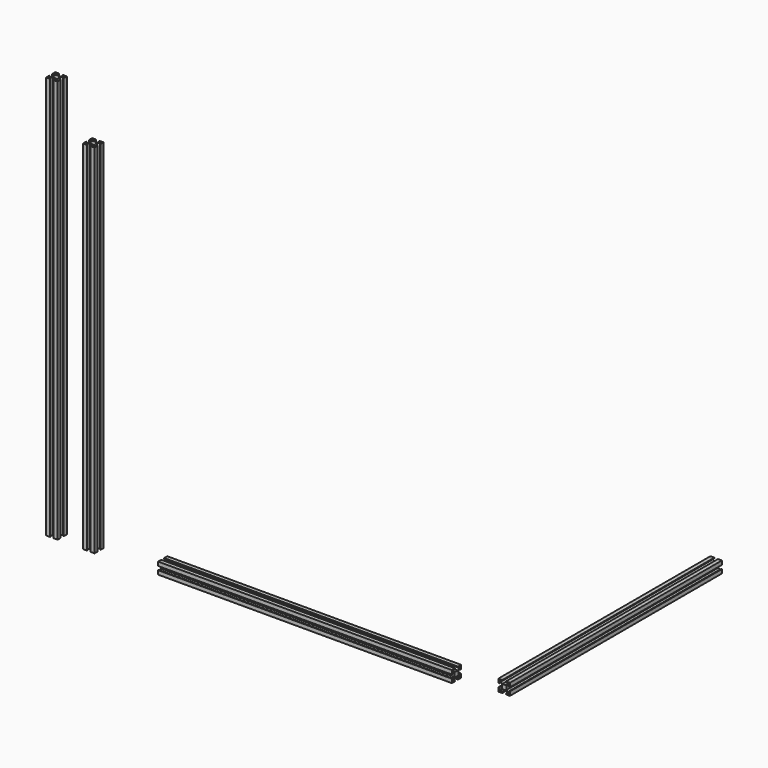
from build123d import *

# Parameters (mm, degrees)
F0_W     = 20
F0_H     = 700
F1_DEPTH = 20
F0_W_2   = 510
F0_H_2   = 20
F0_H_3   = 620
F2_DEPTH = 460
F4_DEPTH = 620
F6_DEPTH = 700
F8_DEPTH = 510


# Not quite as in the source:
# - a feature names something its author has since deleted; it is built from what else it names


with BuildPart() as f1:
    # F0 (on Front) → F1 (new body)
    with BuildSketch(Plane.XZ):
        with Locations((-54.1069640219, 280.5815398693)):
            Rectangle(F0_W, F0_H)
    extrude(amount=F1_DEPTH)

    # F5 (on face) → F6 (cut, through all)
    with BuildSketch(Plane.XY.offset(630.5815398693)):
        Polygon((-62.7069640219, -6.8), (-64.1069640219, -6.8), (-64.1069640219, -13.2), (-62.7069640219, -13.2), (-62.7069640219, -17.6100505063), (-58.1069640219, -13.0100505063), (-58.1069640219, -10), (-58.1069640219, -6.9899494937), (-62.7069640219, -2.3899494937), align=None)
        Polygon((-50.9069640219, 0), (-57.3069640219, 0), (-57.3069640219, -1.4), (-61.7170145283, -1.4), (-57.1170145283, -6), (-54.1069640219, -6), (-51.0969135156, -6), (-46.4969135156, -1.4), (-50.9069640219, -1.4), align=None)
        Polygon((-44.1069640219, -13.2), (-44.1069640219, -6.8), (-45.5069640219, -6.8), (-45.5069640219, -2.3899494937), (-50.1069640219, -6.9899494937), (-50.1069640219, -10), (-50.1069640219, -13.0100505063), (-45.5069640219, -17.6100505063), (-45.5069640219, -13.2), align=None)
        Polygon((-57.3069640219, -18.6), (-57.3069640219, -20), (-50.9069640219, -20), (-50.9069640219, -18.6), (-46.4969135156, -18.6), (-51.0969135156, -14), (-54.1069640219, -14), (-57.1170145283, -14), (-61.7170145283, -18.6), align=None)
    extrude(amount=-F6_DEPTH, mode=Mode.SUBTRACT)


with BuildPart() as f1b:
    # F0 (on Front) → F1, piece 2 (new body)
    with BuildSketch(Plane.XZ):
        with Locations((385.2474099398, -56.0215914249)):
            Rectangle(F0_W_2, F0_H_2)
    extrude(amount=F1_DEPTH)

    # F7 (on face) → F8 (cut, through all)
    with BuildSketch(Plane(origin=(130.2474099398, 0, 0), x_dir=(0, -1, 0), z_dir=(-1, 0, 0))):
        Polygon((13.2, -46.0215914249), (6.8, -46.0215914249), (6.8, -47.4215914249), (2.3899494937, -47.4215914249), (6.9899494937, -52.0215914249), (10, -52.0215914249), (13.0100505063, -52.0215914249), (17.6100505063, -47.4215914249), (13.2, -47.4215914249), align=None)
        Polygon((20, -59.2215914249), (20, -52.8215914249), (18.6, -52.8215914249), (18.6, -48.4115409186), (14, -53.0115409186), (14, -56.0215914249), (14, -59.0316419313), (18.6, -63.6316419313), (18.6, -59.2215914249), align=None)
        Polygon((6.8, -64.6215914249), (6.8, -66.0215914249), (13.2, -66.0215914249), (13.2, -64.6215914249), (17.6100505063, -64.6215914249), (13.0100505063, -60.0215914249), (10, -60.0215914249), (6.9899494937, -60.0215914249), (2.3899494937, -64.6215914249), align=None)
        Polygon((1.4, -52.8215914249), (0, -52.8215914249), (0, -59.2215914249), (1.4, -59.2215914249), (1.4, -63.6316419313), (6, -59.0316419313), (6, -56.0215914249), (6, -53.0115409186), (1.4, -48.4115409186), align=None)
    extrude(amount=-F8_DEPTH, mode=Mode.SUBTRACT)


with BuildPart() as f1c:
    # F0 (on Front) → F1, piece 3 (new body)
    with BuildSketch(Plane.XZ):
        with Locations((10, 240.5815398693)):
            Rectangle(F0_W, F0_H_3)
    extrude(amount=F1_DEPTH)

    # F3 (on face) → F4 (cut, through all)
    with BuildSketch(Plane.XY.offset(550.5815398693)):
        Polygon((13.2, 0), (6.8, 0), (6.8, -1.4), (2.3899494937, -1.4), (6.9899494937, -6), (10, -6), (13.0100505063, -6), (17.6100505063, -1.4), (13.2, -1.4), align=None)
        Polygon((20, -13.2), (20, -6.8), (18.6, -6.8), (18.6, -2.3899494937), (14, -6.9899494937), (14, -10), (14, -13.0100505063), (18.6, -17.6100505063), (18.6, -13.2), align=None)
        Polygon((6.8, -18.6), (6.8, -20), (13.2, -20), (13.2, -18.6), (17.6100505063, -18.6), (13.0100505063, -14), (10, -14), (6.9899494937, -14), (2.3899494937, -18.6), align=None)
        Polygon((1.4, -6.8), (0, -6.8), (0, -13.2), (1.4, -13.2), (1.4, -17.6100505063), (6, -13.0100505063), (6, -10), (6, -6.9899494937), (1.4, -2.3899494937), align=None)
    extrude(amount=-F4_DEPTH, mode=Mode.SUBTRACT)


with BuildPart() as f2:
    # F0 (on Front) → F2 (new body)
    with BuildSketch(Plane.XZ):
        Polygon((705.0956487656, -59.2215914249), (705.0956487656, -66.0215914249), (711.8956487656, -66.0215914249), (711.8956487656, -64.6215914249), (707.4855982592, -64.6215914249), (712.0855982592, -60.0215914249), (715.0956487656, -60.0215914249), (718.1056992719, -60.0215914249), (722.7056992719, -64.6215914249), (718.2956487656, -64.6215914249), (718.2956487656, -66.0215914249), (725.0956487656, -66.0215914249), (725.0956487656, -59.2215914249), (723.6956487656, -59.2215914249), (723.6956487656, -63.6316419313), (719.0956487656, -59.0316419313), (719.0956487656, -56.0215914249), (719.0956487656, -53.0115409186), (723.6956487656, -48.4115409186), (723.6956487656, -52.8215914249), (725.0956487656, -52.8215914249), (725.0956487656, -46.0215914249), (718.2956487656, -46.0215914249), (718.2956487656, -47.4215914249), (722.7056992719, -47.4215914249), (718.1056992719, -52.0215914249), (715.0956487656, -52.0215914249), (712.0855982592, -52.0215914249), (707.4855982592, -47.4215914249), (711.8956487656, -47.4215914249), (711.8956487656, -46.0215914249), (705.0956487656, -46.0215914249), (705.0956487656, -52.8215914249), (706.4956487656, -52.8215914249), (706.4956487656, -48.4115409186), (711.0956487656, -53.0115409186), (711.0956487656, -56.0215914249), (711.0956487656, -59.0316419313), (706.4956487656, -63.6316419313), (706.4956487656, -59.2215914249), align=None)
    extrude(amount=-F2_DEPTH)


solid = Compound([f1.part, f1b.part, f1c.part, f2.part])
